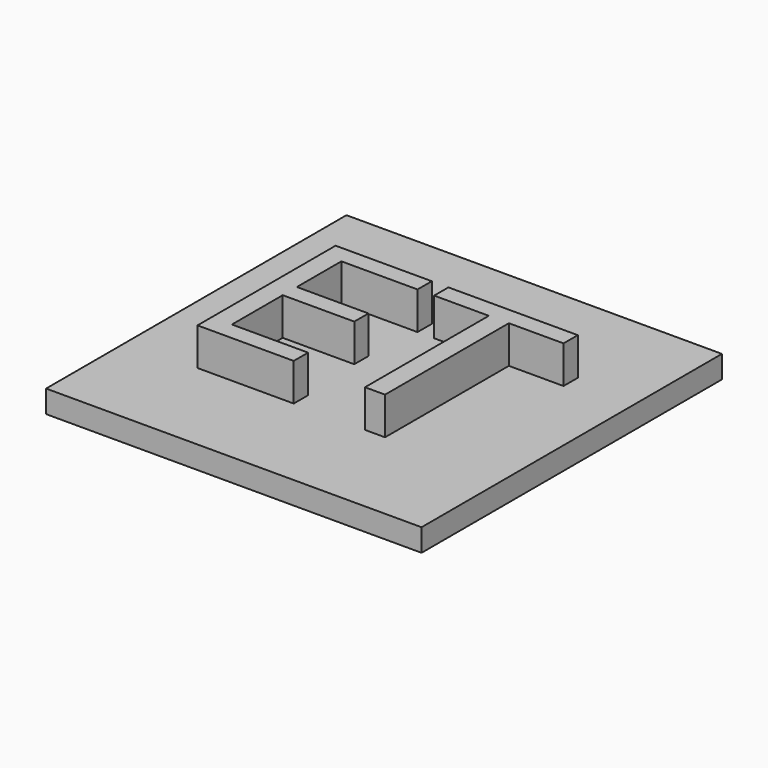
from build123d import *

# Parameters (mm, degrees)
F0_W         = 20
F0_H         = 20
F1_DEPTH     = 1.2
F2_TEXT_SIZE = 12.8772635815
F3_DEPTH     = 2


# Not quite as in the source:
# - Text() gives the source's letters only with a copy of the font that has no kerning and outlines rounded to 1/6400 em; it was checked with that copy


with BuildPart() as f1:
    # F0 (on Top) → F1 (new body)
    with BuildSketch(Plane.XY):
        Rectangle(F0_W, F0_H)
    extrude(amount=F1_DEPTH)

    # F2 (on face) → F3 (join)
    with BuildSketch(Plane.XY.offset(1.2)):
        with Locations((-7.5, -4.6216297787)):
            Text('ET', F2_TEXT_SIZE, font='Open Sans', text_align=(TextAlign.LEFT, TextAlign.BOTTOM))
    extrude(amount=F3_DEPTH)


solid = f1.part
